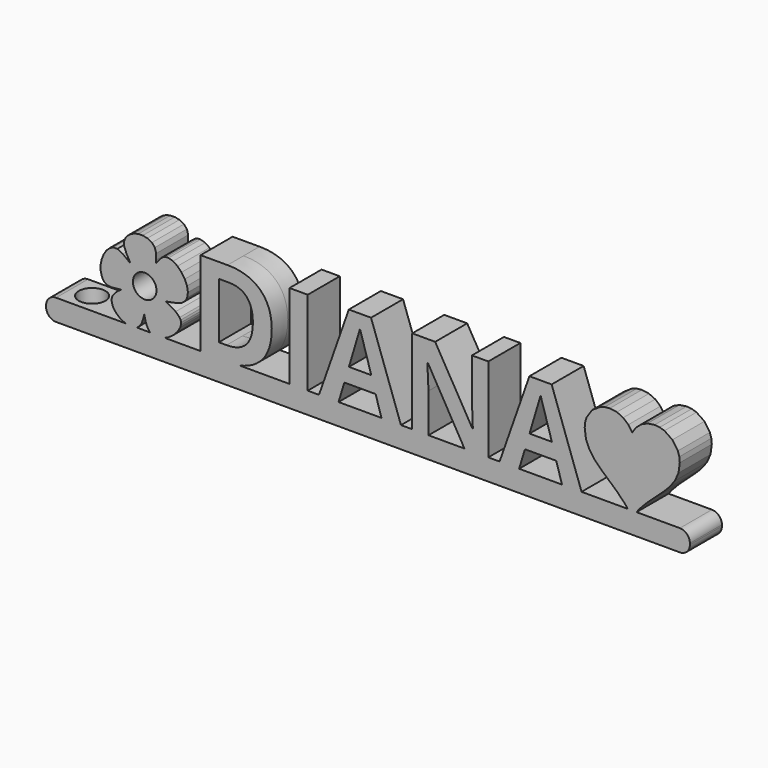
from build123d import *

# Parameters (mm, degrees)
F0_R         = 1.7660260944
F0_TEXT_SIZE = 18.0103437785
F1_DEPTH     = 3
F2_W         = 89
F2_H         = 6
F3_DEPTH     = 0.2
F4_DEPTH     = 3
F5_W         = 6
F5_H         = 3.2
F6_DEPTH     = 7.5
F7_R         = 1.5
F8_R         = 2
F9_DEPTH     = 4
F10_R        = 1.5


# Not quite as in the source:
# - Text() gives the source's letters only with a copy of the font that has no kerning and outlines rounded to 1/6400 em; it was checked with that copy


with BuildPart() as f1:
    # F0 (on Front) → F1 (new body, symmetric)
    with BuildSketch(Plane.XZ):
        Polygon((-9.8962181259, -0.0299609487), (-9.3093152472, 0.0995427735), (-8.5310452338, 0.4643787281), (-7.7886221935, 1.0156229815), (-7.1753136859, 1.6703047867), (-6.7844076966, 2.345448762), (-6.6844409889, 2.697736103), (-6.6652413988, 3.0240118702), (-6.7312263226, 3.3305926174), (-6.8868132072, 3.6238062576), (-7.4844896445, 4.1953846804), (-8.4936258745, 4.789299945), (-8.9274018823, 5.0567831788), (-8.4181052429, 5.1580766137), (-7.3131137554, 5.3695361907), (-6.5480905692, 5.6521941874), (-6.0523445823, 6.043851435), (-5.7552051187, 6.5823041299), (-5.6420905942, 7.3346827833), (-5.7751165223, 8.1369112107), (-6.1089634595, 8.9328581362), (-6.5983028952, 9.6663968681), (-7.1978267956, 10.281407439), (-7.8622157172, 10.7217585729), (-8.546147975, 10.9313258196), (-8.8812811082, 10.9320270148), (-9.2043064176, 10.8539824368), (-9.6469000392, 10.5612860557), (-10.1400767255, 9.9810366231), (-10.4508130024, 9.5801644376), (-10.4068223535, 10.0271686751), (-10.3916193646, 10.9311557532), (-10.598433195, 11.6324207168), (-11.0363252865, 12.1480644274), (-11.7143548393, 12.4951945719), (-12.3982545289, 12.6383143795), (-13.0712303381, 12.6247535348), (-13.7032208938, 12.4733707309), (-14.2641853, 12.2030313855), (-14.7240621838, 11.8325941916), (-15.0528129411, 11.3809291004), (-15.2203761991, 10.8668948051), (-15.1967042361, 10.3093544817), (-14.8286469794, 9.4077545862), (-14.3529716358, 8.5454741101), (-14.2906102139, 8.4004774316), (-14.4811582303, 8.5293860258), (-15.3946726039, 9.2300894295), (-16.21802192, 9.6332437342), (-16.8030362894, 9.634121823), (-17.3568401554, 9.3699870508), (-17.8525159958, 8.8932532172), (-18.2631576982, 8.2563454299), (-18.5618432066, 7.5116797807), (-18.7216618753, 6.7116836696), (-18.7156984739, 5.9087754295), (-18.5170445979, 5.1553756349), (-18.2008868091, 4.6439944488), (-17.7512302174, 4.3560670179), (-17.1086136552, 4.2712956407), (-16.2135760559, 4.3694053341), (-15.7044514474, 4.4302814773), (-15.6696932647, 4.4000047008), (-15.7790195709, 4.3290260096), (-16.1651405309, 4.0708069691), (-16.5523139664, 3.7127982689), (-16.8671052824, 3.3322639471), (-17.0360798838, 3.0064680418), (-17.0831036318, 2.6043628391), (-17.0239245605, 2.1921008316), (-16.867618816, 1.7819255621), (-16.6232807801, 1.3860941234), (-16.3000002503, 1.0168545414), (-15.9068693162, 0.6864593752), (-15.4529754831, 0.4071521172), (-14.9474063577, 0.1911989779), (-14.4397479673, 0.0570083052), (-13.9840845603, 0.0188926715), (-13.5797273957, 0.0772799851), (-13.2259605822, 0.2326232662), (-12.9220907946, 0.485341356), (-12.6674066752, 0.8358849825), (-12.4612081239, 1.2846821047), (-12.3027905578, 1.8321743328), (-12.1879723822, 2.2557758958), (-12.1309056827, 2.0998483864), (-12.0112204133, 1.5291342486), (-11.8237778137, 0.9902805659), (-11.5954117235, 0.5466869075), (-11.3529559319, 0.2617414835), (-10.9521058183, 0.053843468), (-10.4551700276, -0.0442881949), align=None)
        with Locations((-12.1185852993, 6.0541479067)):
            Circle(F0_R, mode=Mode.SUBTRACT)
        Polygon((58.6602663837, 12.4433699982), (57.5992463837, 12.5970599982), (56.8406363837, 12.5204799982), (56.1338363837, 12.3008699982), (54.9364963837, 11.4933499982), (54.1288763837, 10.2961199982), (53.9092263837, 9.5893599982), (53.8326363837, 8.8307599982), (54.0211563837, 7.3860999982), (54.5418963837, 6.1597099982), (55.3276463837, 5.0814099982), (56.3111763837, 4.0810299982), (58.6080263837, 2.0250499982), (59.7926163837, 0.8247399982), (60.9156063837, -0.5860800018), (60.9598863837, -0.6500000018), (61.0029163837, -0.5851400018), (62.0808263837, 0.8234499982), (63.2441263837, 2.0333299982), (65.5477963837, 4.1212499982), (66.5485863837, 5.1327499982), (67.3535863837, 6.2116199982), (67.8899763837, 7.4226699982), (68.0849563837, 8.8307599982), (68.0083763837, 9.5893599982), (67.7887663837, 10.2961199982), (66.9812463837, 11.4933499982), (65.7840163837, 12.3008699982), (65.0772463837, 12.5204799982), (64.3186563837, 12.5970599982), (63.2576363837, 12.4433699982), (62.3165663837, 12.0123599982), (61.5366163837, 11.3491699982), (60.9589463837, 10.4989199982), (60.3812863837, 11.3491699982), (59.6013363837, 12.0123599982), align=None)
        with Locations((-5.3603742014, 0)):
            Text('DIANA', F0_TEXT_SIZE, font='Open Sans', font_style=FontStyle.BOLD, text_align=(TextAlign.LEFT, TextAlign.BOTTOM))
    extrude(amount=F1_DEPTH, both=True)



with BuildPart() as f3:
    # F2 (on Top) → F3 (new body)
    with BuildSketch(Plane.XY):
        with Locations((25.1, 0)):
            Rectangle(F2_W, F2_H)
    extrude(amount=F3_DEPTH)


with BuildPart() as f4:
    # F4 (new): a face of the model
    f4_faces = [f3.part.faces().sort_by_distance(p)[0] for p in [
        (25.1, 0, 0),
    ]]
    extrude(f4_faces, amount=F4_DEPTH)


with BuildPart() as f1_1:
    add(f1.part)

    add(f3.part)  # F6 merges F3

    add(f4.part)  # F6 merges F4
    # F5 (on face) → F6 (join)
    with BuildSketch(Plane(origin=(-19.4, 0, 0), x_dir=(0, -1, 0), z_dir=(-1, 0, 0))):
        with Locations((0, -1.4)):
            Rectangle(F5_W, F5_H)
    extrude(amount=F6_DEPTH)

    # F7
    f7_edges = [f1_1.edges().sort_by_distance(p)[0] for p in [
        (-26.9, 0, -3),
        (-26.9, 0, 0.2),
        (69.6, 0, -3),
    ]]
    fillet(f7_edges, radius=F7_R)

    # F8 (on face) → F9 (cut)
    with BuildSketch(Plane.XY.offset(0.2)):
        with Locations((-22.4, 0)):
            Circle(F8_R)
    extrude(amount=-F9_DEPTH, mode=Mode.SUBTRACT)

    # F10
    f10_edges = [f1_1.edges().sort_by_distance(p)[0] for p in [
        (69.6, 0, 0.2),
    ]]
    fillet(f10_edges, radius=F10_R)


solid = f1_1.part
